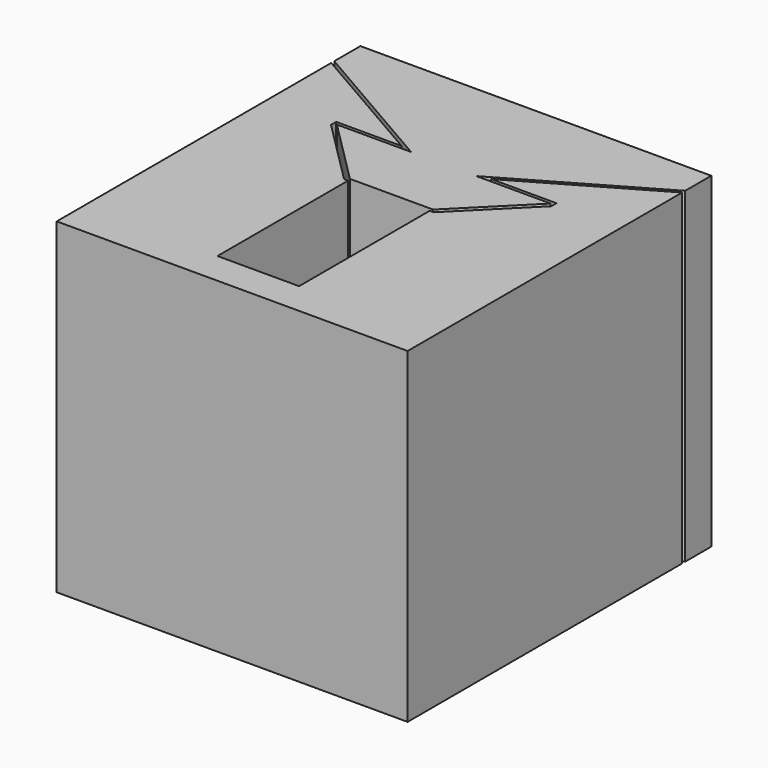
from build123d import *

# Parameters (mm, degrees)
F1_DEPTH  = 5
F2_SIZE   = 1.99999
F2_2_SIZE = 1.99999


# Not quite as in the source:
# - a fillet or chamfer is up to 0.001 mm smaller than in the source, because OpenCascade refuses the exact size


with BuildPart() as f1:
    # F0 (on Top) → F1 (new body, symmetric)
    with BuildSketch(Plane.XY):
        Polygon((-3.8368740493, -3.3047820088), (-3.8368740493, -9.3047820088), (6.9095361123, -9.3047820088), (6.9095361123, -3.3047820088), (4.9095361123, -3.3047820088), (2.7863310315, -3.3047820088), (2.7863310315, -8.3047820088), (0.2863310315, -8.3047820088), (0.2863310315, -3.3047820088), (-1.8368740493, -3.3047820088), align=None)
        Polygon((4.9095361123, -3.3047820088), (6.9095361123, -3.3047820088), (6.9095361123, 1.204619068), (2.9095361123, -1.1047820088), (4.9095361123, -1.1047820088), align=None)
        Polygon((-3.8368740493, 1.204619068), (-3.8368740493, -3.3047820088), (-1.8368740493, -3.3047820088), (-1.8368740493, -1.1047820088), (0.1631259507, -1.1047820088), align=None)
    extrude(amount=F1_DEPTH, both=True)

    # F2 (size 2 in the source; OpenCascade refuses exactly that, so slightly less here)
    f2_edges = [f1.edges().sort_by_distance(p)[0] for p in [
        (4.909536, -3.304782, 0),
        (-1.836874, -3.304782, 0),
    ]]
    chamfer(f2_edges, length=F2_SIZE)


with BuildPart() as f1b:
    # F0 (on Top) → F1, piece 2 (new body, symmetric)
    with BuildSketch(Plane.XY):
        Polygon((4.8095361123, -3.2047820088), (4.8095361123, -1.2047820088), (2.5363310315, -1.2047820088), (6.9095361123, 1.3200891218), (6.9095361123, 2.3200891218), (1.5363310315, 2.3200891218), (-3.8368740493, 2.3200891218), (-3.8368740493, 1.3200891218), (0.5363310315, -1.2047820088), (-1.7368740493, -1.2047820088), (-1.7368740493, -3.2047820088), (1.5363310315, -3.2047820088), align=None)
    extrude(amount=F1_DEPTH, both=True)

    # F2#2 (size 2 in the source; OpenCascade refuses exactly that, so slightly less here)
    f2_2_edges = [f1b.edges().sort_by_distance(p)[0] for p in [
        (4.809536, -3.204782, 0),
        (-1.736874, -3.204782, 0),
    ]]
    chamfer(f2_2_edges, length=F2_2_SIZE)


solid = Compound([f1.part, f1b.part])
